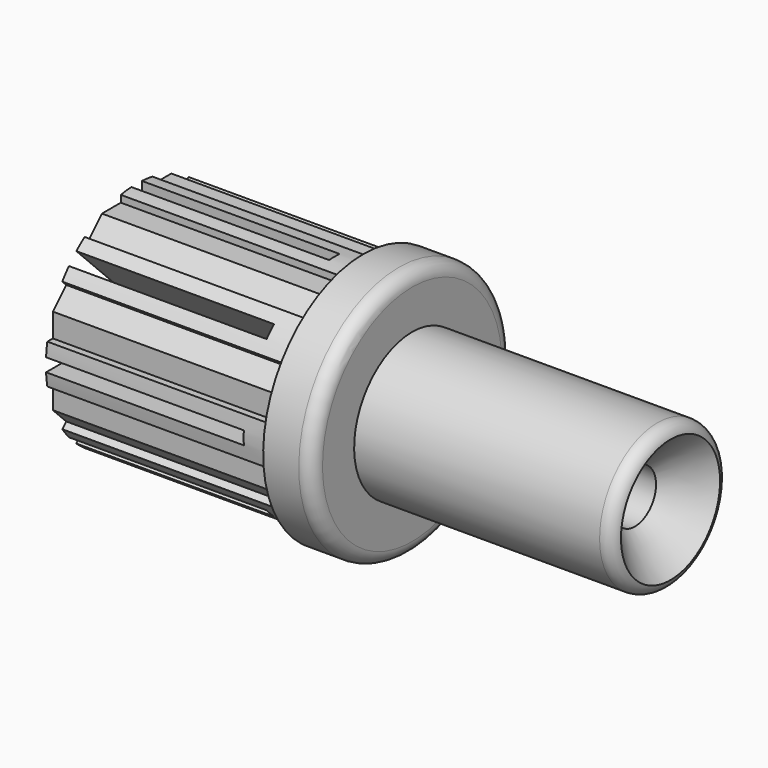
from build123d import *

# Parameters (mm, degrees)
F5_W            = 1
F5_H            = 9
F6_DEPTH        = 15
F6_COPIES_COUNT = 8
F7_W            = 1.7910775183
F7_H            = 2
F8_DEPTH        = 17.2
F8_COPIES_COUNT = 8


# Not quite as in the source:
# - a fillet or chamfer that OpenCascade refuses, or shapes differently, is made with other operations: its cross-section is extruded or revolved along the edge and cut away or added
# - a pattern or mirror of a feature is missing from the dataset's text; its kind, count and spacing are read off the source's solid


with BuildPart() as f2:
    # F0 (on Front) → F2 (revolve)
    with BuildSketch(Plane.XZ):
        Polygon((-17.2, 0), (23.3, 0), (23.3, 5.5), (3.7, 5.5), (3.7, 9.5), (0, 9.5), (0, 8.6), (-17.2, 8.6), align=None)
    revolve(axis=Axis((3.6722049117, 0, 0), (1, 0, 0)))

    # F3 (on Front) → F4 (revolve, cut)
    with BuildSketch(Plane.XZ):
        Polygon((-17.2, 0), (23.3, 0), (23.3, 4.7), (20.6, 2), (0, 2), (0, 4), (-2.5, 4), (-2.5, 2), (-17.2, 2), align=None)
    revolve(axis=Axis((3.05, 0, 0), (1, 0, 0)), mode=Mode.SUBTRACT)

    # F5 (on face) → F6 (cut)
    with BuildSketch(Plane(origin=(-17.2, 0, 0), x_dir=(0, -1, 0), z_dir=(-1, 0, 0))):
        with Locations((0, 4.5)):
            Rectangle(F5_W, F5_H)
    f6 = extrude(amount=-F6_DEPTH, mode=Mode.SUBTRACT)

    # F6_copies: F6 ×8 about axis
    f6_copies_axis = Axis((0, 0, 0), (1, 0, 0))
    for i in range(1, F6_COPIES_COUNT):
        add(f6.rotate(f6_copies_axis, i * 360 / F6_COPIES_COUNT), mode=Mode.SUBTRACT)

    # F7 (on face) → F8 (cut, through all)
    with BuildSketch(Plane(origin=(-17.2, 0, 0), x_dir=(0, -1, 0), z_dir=(-1, 0, 0))):
        Polygon((4.7052910807, 9.359577542), (3.2910775183, 7.9453639796), (4.5575605772, 6.6788809207), (5.9717741396, 8.0930944831), align=None)
        with Locations((2.3955387592, 8.9453639796)):
            Rectangle(F7_W, F7_H)
    f8 = extrude(amount=-F8_DEPTH, mode=Mode.SUBTRACT)

    # F8_copies: F8 ×8 about axis
    f8_copies_axis = Axis((0, 0, 0), (1, 0, 0))
    for i in range(1, F8_COPIES_COUNT):
        add(f8.rotate(f8_copies_axis, i * 360 / F8_COPIES_COUNT), mode=Mode.SUBTRACT)

    # F9: fillet of radius 1 on 2 edges, made by hand

    # F9_s1 → F9_t2 (revolve, cut)
    with BuildSketch(Plane.XZ):
        with BuildLine():
            ThreePointArc((23.3, 4.7), (22.9526596349, 5.2745966692), (22.3202041029, 5.5))
            Line((22.3202041029, 5.5), (23.3, 5.5))
            Line((23.3, 5.5), (23.3, 4.7))
        make_face()
    revolve(axis=Axis((23.3, 0, 0), (1, 0, 0)), mode=Mode.SUBTRACT)

    # F9_s3 → F9_t4 (revolve, cut)
    with BuildSketch(Plane.XZ):
        with BuildLine():
            ThreePointArc((2.7, 9.5), (3.4071067812, 9.2071067812), (3.7, 8.5))
            Line((3.7, 8.5), (3.7, 9.5))
            Line((3.7, 9.5), (2.7, 9.5))
        make_face()
    revolve(axis=Axis((3.7, 0, 0), (1, 0, 0)), mode=Mode.SUBTRACT)


solid = f2.part
